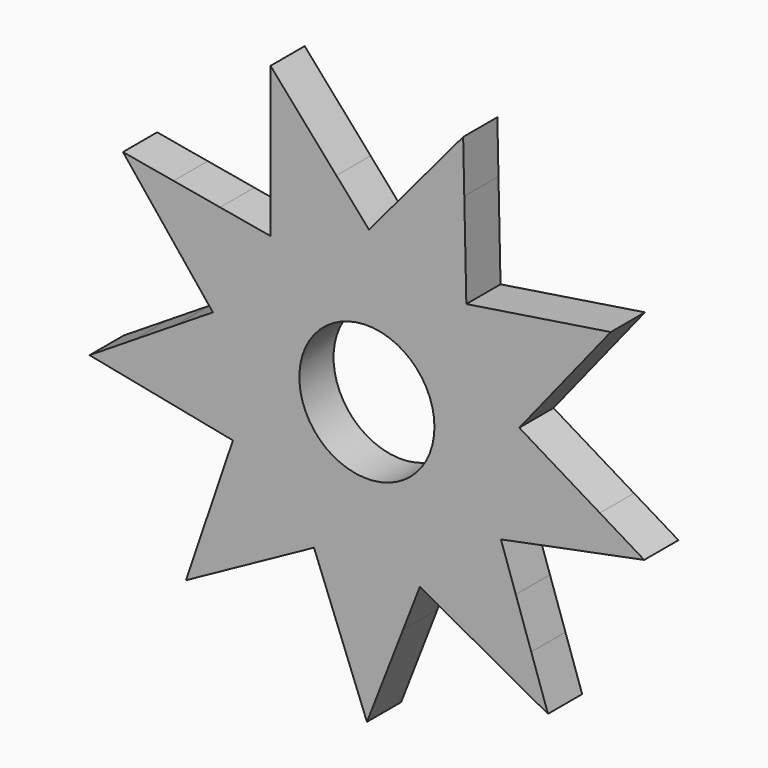
from build123d import *

# Parameters (mm, degrees)
F1_DEPTH = 6.96


# Not quite as in the source:
# - a feature of the source that left no trace in its solid (it failed there, or was rolled back) is left out
# - a feature names something its author has since deleted; it is built from what else it names


with BuildPart() as f1:
    # F0 (on Front) → F1 (new body)
    with BuildSketch(Plane.XZ):
        with BuildLine():
            Line((-4.9618439889, 30.8489073878), (-10.120921757, 36.7311440441))
            ThreePointArc((-10.120921757, 36.7311440441), (-12.9466687362, 35.832858784), (-15.6940034453, 34.7175496811))
            Line((-15.6940034453, 34.7175496811), (-15.6940034453, 27.0180169266))
            ThreePointArc((-15.6940034453, 27.0180169266), (-10.5040439231, 29.4268592285), (-4.9618439889, 30.8489073878))
        make_face()
        with BuildLine():
            ThreePointArc((-15.6940034453, 34.7175496811), (-12.9466687362, 35.832858784), (-10.120921757, 36.7311440441))
            Line((-10.120921757, 36.7311440441), (-15.6940034453, 43.0854164294))
            Line((-15.6940034453, 43.0854164294), (-15.6940034453, 34.7175496811))
        make_face()
        with BuildLine():
            Line((0.3367577987, 24.8075893339), (-4.9618439889, 30.8489073878))
            ThreePointArc((-4.9618439889, 30.8489073878), (-10.5040439231, 29.4268592285), (-15.6940034453, 27.0180169266))
            Line((-15.6940034453, 27.0180169266), (-15.6940034453, 18.6877066835))
            Line((-15.6940034453, 18.6877066835), (-6.1980460207, 17.0157598588))
            Line((-6.1980460207, 17.0157598588), (0.3367577987, 24.8075893339))
        make_face()
        with BuildLine():
            Line((5.349116457, 30.7841182417), (0.3367577987, 24.8075893339))
            Line((0.3367577987, 24.8075893339), (-6.1980460207, 17.0157598588))
            Line((-6.1980460207, 17.0157598588), (-15.6940034453, 18.6877066835))
            Line((-15.6940034453, 18.6877066835), (-15.6940034453, 10.6181583146))
            Line((-15.6940034453, 10.6181583146), (-25.0790561702, 4.6957263488))
            Line((-25.0790561702, 4.6957263488), (-18.6598426779, -3.2950419376))
            Line((-18.6598426779, -3.2950419376), (-21.8185465433, -12.6017368372))
            Line((-21.8185465433, -12.6017368372), (-12.1835113634, -14.5123768209))
            Line((-12.1835113634, -14.5123768209), (-8.6159947437, -23.6812639315))
            Line((-8.6159947437, -23.6812639315), (0, -18.9485363587))
            Line((0, -18.9485363587), (8.6238023794, -23.6784231328))
            Line((8.6238023794, -23.6784231328), (12.1835113634, -14.5123768209))
            Line((12.1835113634, -14.5123768209), (21.8258896669, -12.5939120432))
            Line((21.8258896669, -12.5939120432), (18.6614871852, -3.2857154732))
            Line((18.6614871852, -3.2857154732), (24.8148121143, 4.3819151105))
            Line((24.8148121143, 4.3819151105), (29.5186280009, 10.2433189804))
            Line((29.5186280009, 10.2433189804), (34.4156358122, 16.3454584408))
            Line((34.4156358122, 16.3454584408), (39.7056170429, 22.9372803158))
            Line((39.7056170429, 22.9372803158), (16.1926081875, 19.3073954844))
            Line((16.1926081875, 19.3073954844), (15.85724841, 34.6432918884))
            ThreePointArc((15.85724841, 34.6432918884), (14.4513233415, 35.2529325543), (13.0220201926, 35.8055441252))
            Line((13.0220201926, 35.8055441252), (10.6792184181, 29.3637408511))
            ThreePointArc((10.6792184181, 29.3637408511), (8.0455731741, 30.1917825756), (5.349116457, 30.7841182417))
        make_face()
        with BuildLine():
            ThreePointArc((3.7596383758, 10.3375586713), (9.0098840762, 6.3104666177), (11, 0))
            ThreePointArc((11, 0), (-9.0098840762, -6.3104666177), (3.7596383758, 10.3375586713))
        make_face(mode=Mode.SUBTRACT)
        with BuildLine():
            Line((-15.6940034453, 10.6181583146), (-15.6940034453, 18.6877066835))
            Line((-15.6940034453, 18.6877066835), (-23.8953753875, 20.1317167147))
            ThreePointArc((-23.8953753875, 20.1317167147), (-27.1646586752, 15.4387921111), (-29.52374385, 10.2285645068))
            Line((-29.52374385, 10.2285645068), (-25.0790561702, 4.6957263488))
            Line((-25.0790561702, 4.6957263488), (-15.6940034453, 10.6181583146))
        make_face()
        with BuildLine():
            Line((10.2959158336, 36.6824769767), (5.349116457, 30.7841182417))
            ThreePointArc((5.349116457, 30.7841182417), (8.0455731741, 30.1917825756), (10.6792184181, 29.3637408511))
            Line((10.6792184181, 29.3637408511), (13.0220201926, 35.8055441252))
            ThreePointArc((13.0220201926, 35.8055441252), (11.6672099465, 36.2696320916), (10.2959158336, 36.6824769767))
        make_face()
        with BuildLine():
            ThreePointArc((-29.52374385, 10.2285645068), (-27.1646586752, 15.4387921111), (-23.8953753875, 20.1317167147))
            Line((-23.8953753875, 20.1317167147), (-31.476903581, 21.4665912747))
            Line((-31.476903581, 21.4665912747), (-39.7170759686, 22.9174328742))
            Line((-39.7170759686, 22.9174328742), (-29.52374385, 10.2285645068))
        make_face()
        with BuildLine():
            Line((15.6724677094, 43.0932547963), (10.2959158336, 36.6824769767))
            ThreePointArc((10.2959158336, 36.6824769767), (11.6672099465, 36.2696320916), (13.0220201926, 35.8055441252))
            Line((13.0220201926, 35.8055441252), (15.6724677094, 43.0932547963))
        make_face()
        with BuildLine():
            Line((-18.6598426779, -3.2950419376), (-25.0790561702, 4.6957263488))
            Line((-25.0790561702, 4.6957263488), (-31.2348698324, 0.8111037816))
            ThreePointArc((-31.2348698324, 0.8111037816), (-30.7987467244, -5.2642362214), (-29.1922235992, -11.139527105))
            Line((-29.1922235992, -11.139527105), (-21.8185465433, -12.6017368372))
            Line((-21.8185465433, -12.6017368372), (-18.6598426779, -3.2950419376))
        make_face()
        with BuildLine():
            Line((15.85724841, 34.6432918884), (15.6724677094, 43.0932547963))
            Line((15.6724677094, 43.0932547963), (13.0220201926, 35.8055441252))
            ThreePointArc((13.0220201926, 35.8055441252), (14.4513233415, 35.2529325543), (15.85724841, 34.6432918884))
        make_face()
        with BuildLine():
            ThreePointArc((-29.1922235992, -11.139527105), (-30.7987467244, -5.2642362214), (-31.2348698324, 0.8111037816))
            Line((-31.2348698324, 0.8111037816), (-37.9458459601, -3.4238537307))
            ThreePointArc((-37.9458459601, -3.4238537307), (-37.5339500378, -6.54313339), (-36.8660833418, -9.6177907563))
            Line((-36.8660833418, -9.6177907563), (-29.1922235992, -11.139527105))
        make_face()
        with BuildLine():
            Line((-12.1835113634, -14.5123768209), (-21.8185465433, -12.6017368372))
            Line((-21.8185465433, -12.6017368372), (-24.2350154824, -19.7215366379))
            ThreePointArc((-24.2350154824, -19.7215366379), (-20.078672611, -23.9399642642), (-15.2010519849, -27.2984065715))
            Line((-15.2010519849, -27.2984065715), (-8.6159947437, -23.6812639315))
            Line((-8.6159947437, -23.6812639315), (-12.1835113634, -14.5123768209))
        make_face()
        with BuildLine():
            ThreePointArc((-36.8660833418, -9.6177907563), (-37.5339500378, -6.54313339), (-37.9458459601, -3.4238537307))
            Line((-37.9458459601, -3.4238537307), (-45.15608724, -7.9738722218))
            Line((-45.15608724, -7.9738722218), (-36.8660833418, -9.6177907563))
        make_face()
        with BuildLine():
            ThreePointArc((-15.2010519849, -27.2984065715), (-20.078672611, -23.9399642642), (-24.2350154824, -19.7215366379))
            Line((-24.2350154824, -19.7215366379), (-26.7496429738, -27.1305473733))
            ThreePointArc((-26.7496429738, -27.1305473733), (-24.4831574997, -29.1922078446), (-22.0583421712, -31.0650855569))
            Line((-22.0583421712, -31.0650855569), (-15.2010519849, -27.2984065715))
        make_face()
        with BuildLine():
            ThreePointArc((-22.0583421712, -31.0650855569), (-24.4831574997, -29.1922078446), (-26.7496429738, -27.1305473733))
            Line((-26.7496429738, -27.1305473733), (-29.4660634378, -35.1341138854))
            Line((-29.4660634378, -35.1341138854), (-22.0583421712, -31.0650855569))
        make_face()
        with BuildLine():
            Line((0, -18.9485363587), (-8.6159947437, -23.6812639315))
            Line((-8.6159947437, -23.6812639315), (-5.8908957162, -30.6850506021))
            ThreePointArc((-5.8908957162, -30.6850506021), (0.0065066962, -31.2453987085), (5.9036752179, -30.6825944423))
            Line((5.9036752179, -30.6825944423), (8.6238023794, -23.6784231328))
            Line((8.6238023794, -23.6784231328), (0, -18.9485363587))
        make_face()
        with BuildLine():
            ThreePointArc((5.9036752179, -30.6825944423), (0.0065066962, -31.2453987085), (-5.8908957162, -30.6850506021))
            Line((-5.8908957162, -30.6850506021), (-3.0535035766, -37.9774421981))
            Line((-3.0535035766, -37.9774421981), (0.0114589257, -45.8547131899))
            Line((0.0114589257, -45.8547131899), (5.9036752179, -30.6825944423))
        make_face()
        with BuildLine():
            Line((12.1835113634, -14.5123768209), (8.6238023794, -23.6784231328))
            Line((8.6238023794, -23.6784231328), (15.2124188317, -27.2920738691))
            ThreePointArc((15.2124188317, -27.2920738691), (20.0896378001, -23.930763378), (24.2448691352, -19.7094216914))
            Line((24.2448691352, -19.7094216914), (21.8258896669, -12.5939120432))
            Line((21.8258896669, -12.5939120432), (12.1835113634, -14.5123768209))
        make_face()
        with BuildLine():
            Line((31.2416193325, 0.4860085148), (24.8148121143, 4.3819151105))
            Line((24.8148121143, 4.3819151105), (18.6614871852, -3.2857154732))
            Line((18.6614871852, -3.2857154732), (21.8258896669, -12.5939120432))
            Line((21.8258896669, -12.5939120432), (29.1968594713, -11.1273707499))
            ThreePointArc((29.1968594713, -11.1273707499), (30.7720664648, -5.418017006), (31.2416193325, 0.4860085148))
        make_face()
        with BuildLine():
            ThreePointArc((24.2448691352, -19.7094216914), (20.0896378001, -23.930763378), (15.2124188317, -27.2920738691))
            Line((15.2124188317, -27.2920738691), (22.0728280834, -31.0547944833))
            ThreePointArc((22.0728280834, -31.0547944833), (24.4972570827, -29.1803768897), (26.7631992818, -27.117174709))
            Line((26.7631992818, -27.117174709), (24.2448691352, -19.7094216914))
        make_face()
        with BuildLine():
            Line((37.9323840026, -3.569908105), (31.2416193325, 0.4860085148))
            ThreePointArc((31.2416193325, 0.4860085148), (30.7720664648, -5.418017006), (29.1968594713, -11.1273707499))
            Line((29.1968594713, -11.1273707499), (36.8705647308, -9.6005966708))
            ThreePointArc((36.8705647308, -9.6005966708), (37.5228275313, -6.6066189578), (37.9323840026, -3.569908105))
        make_face()
        with BuildLine():
            ThreePointArc((26.7631992818, -27.117174709), (24.4972570827, -29.1803768897), (22.0728280834, -31.0547944833))
            Line((22.0728280834, -31.0547944833), (29.4836195306, -35.1193825745))
            Line((29.4836195306, -35.1193825745), (26.7631992818, -27.117174709))
        make_face()
        with BuildLine():
            Line((45.1600668832, -7.951302544), (37.9323840026, -3.569908105))
            ThreePointArc((37.9323840026, -3.569908105), (37.5228275313, -6.6066189578), (36.8705647308, -9.6005966708))
            Line((36.8705647308, -9.6005966708), (45.1600668832, -7.951302544))
        make_face()
    extrude(amount=F1_DEPTH)


solid = f1.part
